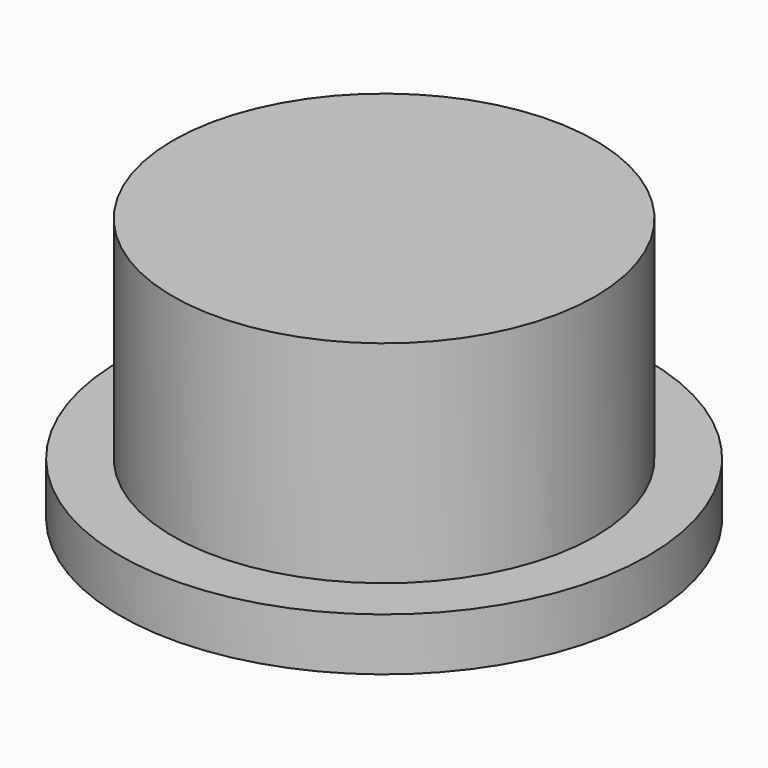
from build123d import *

# Parameters (mm, degrees)
F0_R     = 7.9375
F1_DEPTH = 1.5875
F2_R     = 6.35
F3_DEPTH = 6.35


# Not quite as in the source:
# - a length typed as a fraction of an inch, garbled in the dataset ("3 / 203.2 mm" for 3/8 in), is restored


with BuildPart() as f1:
    # F0 (on Top) → F1 (new body)
    with BuildSketch(Plane.XY):
        Circle(F0_R)
    extrude(amount=F1_DEPTH)

    # F2 (on face) → F3 (join)
    with BuildSketch(Plane.XY.offset(1.5875)):
        Circle(F2_R)
    extrude(amount=F3_DEPTH)


solid = f1.part
